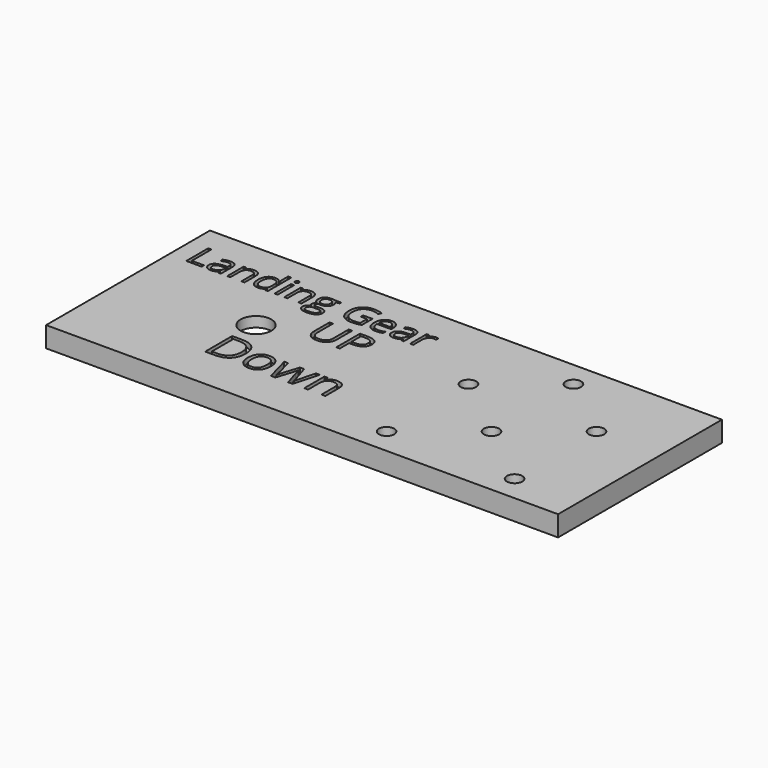
from build123d import *

# Parameters (mm, degrees)
F0_W           = 96
F0_H           = 36
F0_R           = 1.5
F0_R_2         = 3
F1_DEPTH       = 2
F0_W_2         = 100
F0_H_2         = 40
F2_DEPTH       = 4
F3_TEXT_SIZE   = 7.5275463044
F3_TEXT_SIZE_2 = 8.091131167
F3_TEXT_SIZE_3 = 9.2179010001
F4_DEPTH       = 1


# Not quite as in the source:
# - Text() gives the source's letters only with a copy of the font that has no kerning and outlines rounded to 1/6400 em; it was checked with that copy


with BuildPart() as f1:
    # F0 (on Top) → F1 (new body)
    with BuildSketch(Plane.XY):
        Rectangle(F0_W, F0_H)
        with Locations((12.5, -15)):
            Circle(F0_R, mode=Mode.SUBTRACT)
        with Locations((37.5, -15)):
            Circle(F0_R, mode=Mode.SUBTRACT)
        with Locations((25, -5)):
            Circle(F0_R, mode=Mode.SUBTRACT)
        with Locations((-25, 0)):
            Circle(F0_R_2, mode=Mode.SUBTRACT)
        with Locations((12.5, 5)):
            Circle(F0_R, mode=Mode.SUBTRACT)
        with Locations((37.5, 5)):
            Circle(F0_R, mode=Mode.SUBTRACT)
        with Locations((25, 15)):
            Circle(F0_R, mode=Mode.SUBTRACT)
    extrude(amount=-F1_DEPTH)

    # F0 (on Top) → F2 (join)
    with BuildSketch(Plane.XY):
        Rectangle(F0_W_2, F0_H_2)
        Rectangle(F0_W, F0_H, mode=Mode.SUBTRACT)
    extrude(amount=-F2_DEPTH)

    # F3 (on face) → F4 (cut)
    with BuildSketch(Plane.XY):
        with Locations((-47.2741669708, 9.894818314)):
            Text('Landing Gear', F3_TEXT_SIZE, font='Open Sans', text_align=(TextAlign.LEFT, TextAlign.BOTTOM))
        with Locations((-17.5395272672, 1.9339007558)):
            Text('UP', F3_TEXT_SIZE_2, font='Open Sans', text_align=(TextAlign.LEFT, TextAlign.BOTTOM))
        with Locations((-26.4859185554, -11.6756702773)):
            Text('Down', F3_TEXT_SIZE_3, font='Open Sans', text_align=(TextAlign.LEFT, TextAlign.BOTTOM))
    extrude(amount=-F4_DEPTH, mode=Mode.SUBTRACT)


solid = f1.part
